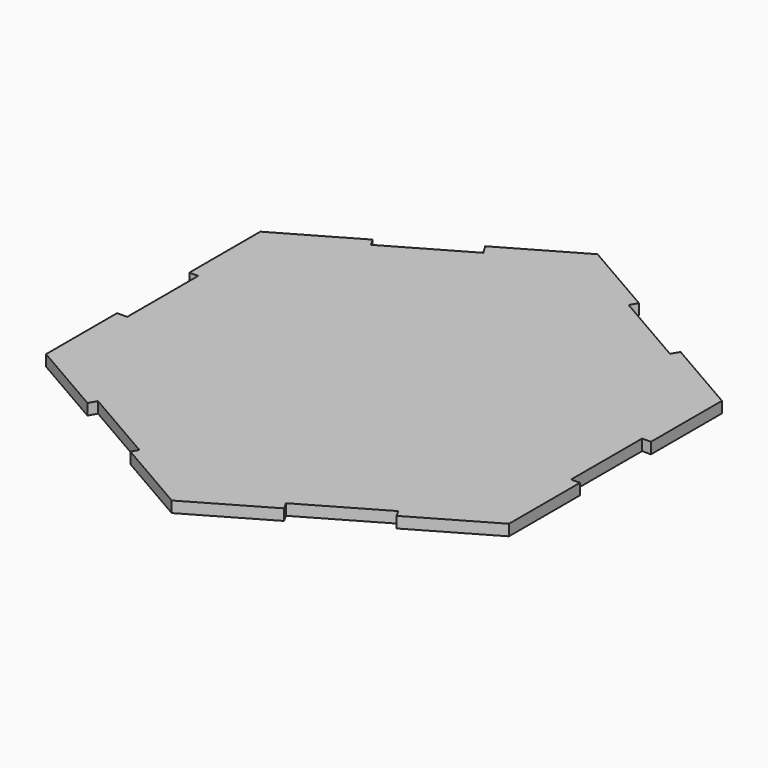
from build123d import *

# Parameters (mm, degrees)
F1_DEPTH = 3.175


# Not quite as in the source:
# - a length typed as a fraction of an inch, garbled in the dataset ("3 / 203.2 mm" for 3/8 in), is restored


with BuildPart() as f1:
    # F0 (on Top) → F1 (new body)
    with BuildSketch(Plane.XY):
        Polygon((-43.6570606842, 50.214136995), (-65.6745214305, 37.5495634813), (-65.6745214305, 12.1495634813), (-63.1345214305, 12.1495634813), (-63.1345214305, -13.2504365187), (-66.0297558966, -13.2504365187), (-66.0297558966, -38.6504365187), (-44.0327106405, -51.3504365187), (-42.7627106405, -49.150731993), (-20.7656653844, -61.850731993), (-21.8444748585, -63.7192848138), (0.1525703977, -76.4192848138), (22.1496156538, -63.7192848138), (20.8796156538, -61.5195802882), (42.8766609099, -48.8195802882), (44.0431281469, -50.8399608081), (66.0401734031, -38.1399608081), (66.0401734031, -12.7399608081), (63.5001734031, -12.7399608081), (63.5001734031, 12.6600391919), (66.0318906401, 12.6600391919), (66.0318906401, 38.0600391919), (44.034845384, 50.7600391919), (42.764845384, 48.5603346662), (20.7678001279, 61.2603346662), (22.0039794371, 63.4014600371), (0.006934181, 76.1014600371), (-22.0105265653, 63.4368865235), (-20.3731425865, 60.6769644341), (-42.3906033328, 48.0123909204), align=None)
    extrude(amount=F1_DEPTH)


solid = f1.part
